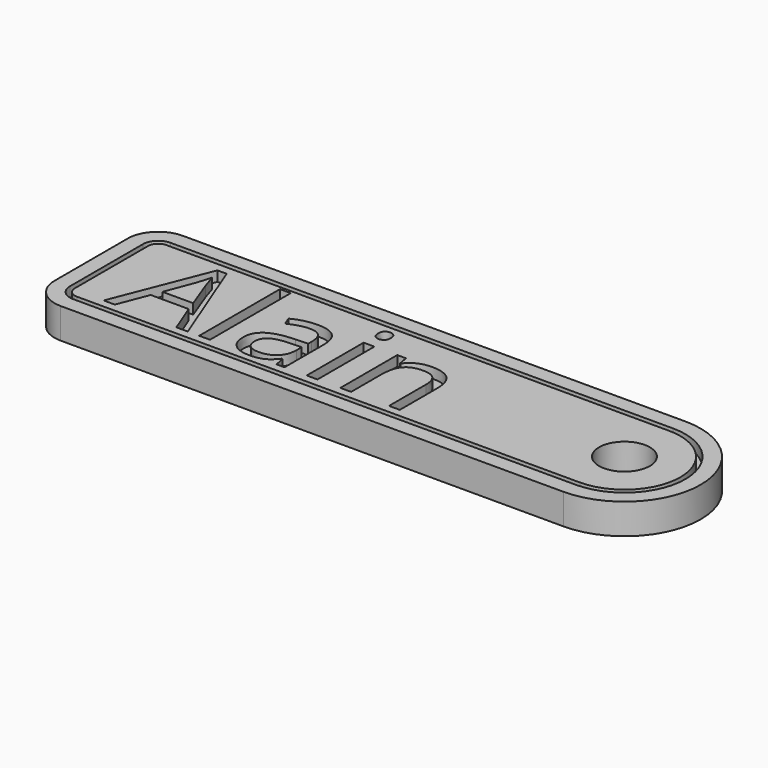
from build123d import *

# Parameters (mm, degrees)
F0_R         = 2.5
F1_DEPTH     = 3
F2_TEXT_SIZE = 13.0834752981
F3_DEPTH     = 1
F6_DEPTH     = 1


# Not quite as in the source:
# - Text() gives the source's letters only with a copy of the font that has no kerning and outlines rounded to 1/6400 em; it was checked with that copy


with BuildPart() as f1:
    # F0 (on Top) → F1 (new body)
    with BuildSketch(Plane.XY):
        with BuildLine():
            Line((22.5, 7.5), (-27, 7.5))
            ThreePointArc((-27, 7.5), (-29.1213203436, 6.6213203436), (-30, 4.5))
            Line((-30, 4.5), (-30, -4.5))
            ThreePointArc((-30, -4.5), (-29.1213203436, -6.6213203436), (-27, -7.5))
            Line((-27, -7.5), (22.5, -7.5))
            ThreePointArc((22.5, -7.5), (30, 0), (22.5, 7.5))
        make_face()
        with Locations((22.5, 0)):
            Circle(F0_R, mode=Mode.SUBTRACT)
    extrude(amount=F1_DEPTH)

    # F2 (on face) → F3 (cut)
    with BuildSketch(Plane.XY.offset(3)):
        with Locations((-25, -4.7100511073)):
            Text('Alain', F2_TEXT_SIZE, font='Open Sans', text_align=(TextAlign.LEFT, TextAlign.BOTTOM))
    extrude(amount=-F3_DEPTH, mode=Mode.SUBTRACT)

    # F5 (on face) → F6 (cut)
    with BuildSketch(Plane.XY.offset(3)):
        with BuildLine():
            Line((22.5, 6), (-27, 6))
            ThreePointArc((-27, 6), (-28.0606601718, 5.5606601718), (-28.5, 4.5))
            Line((-28.5, 4.5), (-28.5, -4.5))
            ThreePointArc((-28.5, -4.5), (-28.0606601718, -5.5606601718), (-27, -6))
            Line((-27, -6), (22.5, -6))
            ThreePointArc((22.5, -6), (28.5, 0), (22.5, 6))
        make_face()
        with BuildLine():
            ThreePointArc((-28, 4.5), (-27.7071067812, 5.2071067812), (-27, 5.5))
            Line((-27, 5.5), (22.5, 5.5))
            ThreePointArc((22.5, 5.5), (28, 0), (22.5, -5.5))
            Line((22.5, -5.5), (-27, -5.5))
            ThreePointArc((-27, -5.5), (-27.7071067812, -5.2071067812), (-28, -4.5))
            Line((-28, -4.5), (-28, 4.5))
        make_face(mode=Mode.SUBTRACT)
    extrude(amount=-F6_DEPTH, mode=Mode.SUBTRACT)


solid = f1.part
